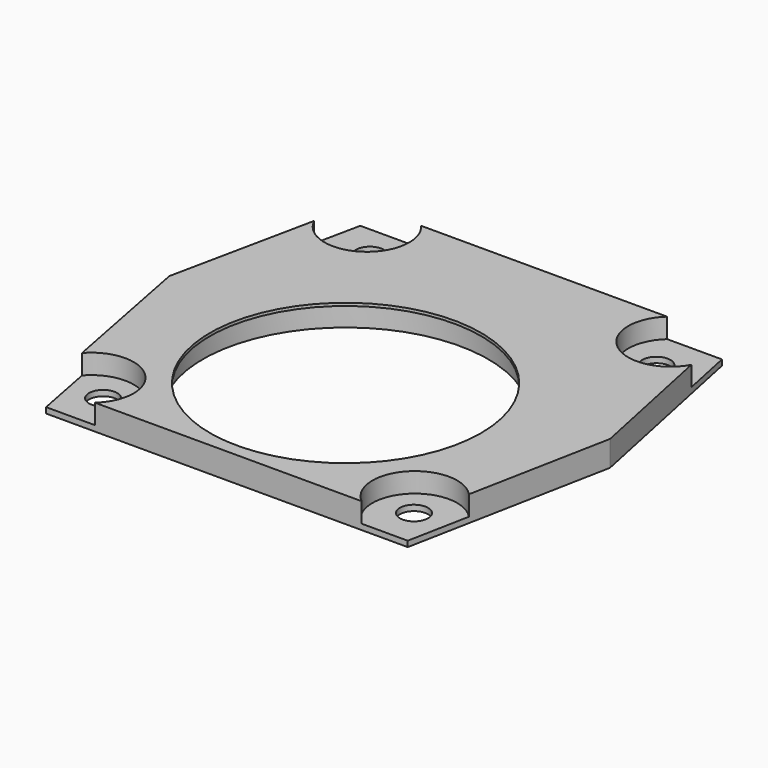
from build123d import *

# Parameters (mm, degrees)
F1_DEPTH = 4.5
F2_R     = 11
F2_R_2   = 24
F3_DEPTH = 50
F2_R_3   = 2.5
F4_DEPTH = 25
F5_DEPTH = 3.5
F6_DEPTH = 2
F7_R     = 25.25
F8_DEPTH = 4


# Not quite as in the source:
# - a feature names something its author has since deleted; it is built from what else it names


with BuildPart() as f1:
    # F0 (on Top) → F1 (new body)
    with BuildSketch(Plane.XY):
        Polygon((-46.0190125704, -8.1893682778), (-110.0190125704, -8.1893682778), (-117.0190125704, -41.6893682778), (-110.0190125704, -77.6893682778), (-46.0190125704, -77.6893682778), (-39.0190125704, -41.6893682778), align=None)
    extrude(amount=F1_DEPTH)

    # F2 (on face) → F3 (cut)
    with BuildSketch(Plane.XY.offset(4.5)):
        with Locations((36.7125935962, -5.1025906342)):
            Circle(F2_R)
        with Locations((63.6127434798, -2.782690585)):
            Circle(F2_R)
        with Locations((-78.0190125704, -51.4393682778)):
            Circle(F2_R_2)
    extrude(amount=-F3_DEPTH, mode=Mode.SUBTRACT)

    # F2 (on face) → F4 (cut)
    with BuildSketch(Plane.XY.offset(4.5)):
        with Locations((-103.5190125704, -14.1893682778)):
            Circle(F2_R_3)
        with Locations((-52.0190125704, -15.1893682778)):
            Circle(F2_R_3)
        with Locations((-105.5190125704, -70.6893682778)):
            Circle(F2_R_3)
        with Locations((-50.5190125704, -70.6893682778)):
            Circle(F2_R_3)
    extrude(amount=-F4_DEPTH, mode=Mode.SUBTRACT)

    # F2 (on face) → F5 (cut)
    with BuildSketch(Plane.XY.offset(4.5)):
        with BuildLine():
            Line((-110.0190125704, -8.1893682778), (-111.7083286904, -16.2739525667))
            ThreePointArc((-111.7083286904, -16.2739525667), (-103.2870621366, -20.4161997132), (-97.4153326836, -13.0950840178))
            ThreePointArc((-97.4153326836, -13.0950840178), (-97.8868841728, -10.4776594188), (-99.2422424253, -8.1893682778))
            Line((-99.2422424253, -8.1893682778), (-110.0190125704, -8.1893682778))
        make_face()
        with Locations((-103.5190125704, -14.1893682778)):
            Circle(F2_R_3, mode=Mode.SUBTRACT)
        with BuildLine():
            Line((-46.0190125704, -8.1893682778), (-55.7181574473, -8.1893682778))
            ThreePointArc((-55.7181574473, -8.1893682778), (-55.3158791173, -19.6211139555), (-44.1027782894, -17.3599180513))
            Line((-44.1027782894, -17.3599180513), (-46.0190125704, -8.1893682778))
        make_face()
        with Locations((-52.0190125704, -15.1893682778)):
            Circle(F2_R_3, mode=Mode.SUBTRACT)
        with BuildLine():
            ThreePointArc((-101.3837870838, -77.6893682778), (-99.5825379735, -75.1790324483), (-98.9461190179, -72.1555815644))
            ThreePointArc((-98.9461190179, -72.1555815644), (-103.7878144934, -65.1424925834), (-112.0616968993, -67.1841345861))
            Line((-112.0616968993, -67.1841345861), (-110.0190125704, -77.6893682778))
            Line((-110.0190125704, -77.6893682778), (-101.3837870838, -77.6893682778))
        make_face()
        with Locations((-105.5190125704, -70.6893682778)):
            Circle(F2_R_3, mode=Mode.SUBTRACT)
        with BuildLine():
            ThreePointArc((-43.9012732129, -66.7981372962), (-54.8452929266, -66.7661737817), (-54.1697108353, -77.6893682778))
            Line((-54.1697108353, -77.6893682778), (-46.0190125704, -77.6893682778))
            Line((-46.0190125704, -77.6893682778), (-43.9012732129, -66.7981372962))
        make_face()
        with Locations((-50.5190125704, -70.6893682778)):
            Circle(F2_R_3, mode=Mode.SUBTRACT)
    extrude(amount=-F5_DEPTH, mode=Mode.SUBTRACT)

    # F2 (on face) → F6 (cut)
    with BuildSketch(Plane.XY.offset(4.5)):
        with Locations((-78.0190125704, -51.4393682778)):
            Circle(F2_R_2)
    extrude(amount=-F6_DEPTH, mode=Mode.SUBTRACT)

    # F7 (on face) → F8 (cut)
    with BuildSketch(Plane(origin=(0, 0, 0), x_dir=(1, 0, 0), z_dir=(0, 0, -1))):
        with Locations((-78.0190125704, 51.4393682778)):
            Circle(F7_R)
    extrude(amount=-F8_DEPTH, mode=Mode.SUBTRACT)


solid = f1.part
